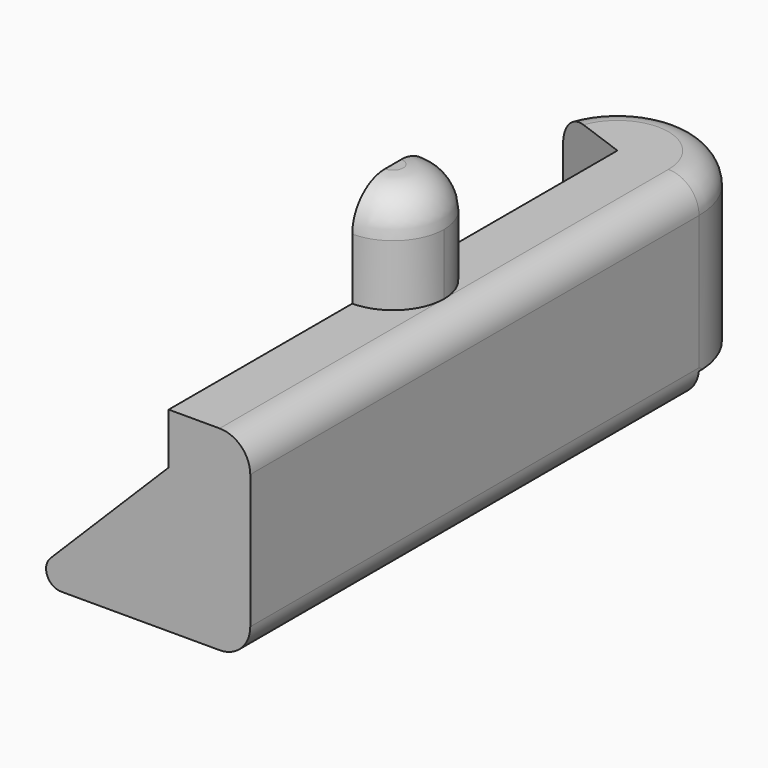
from build123d import *

# Parameters (mm, degrees)
F1_DEPTH      = 5.5
F3_DEPTH      = 1.14554
F4_T1_DEPTH   = 7
F5_R          = 0.15
F7_DEPTH      = 1.5
F7_DEPTH_BACK = 0.8
F8_T2_ANGLE   = 359.64
F9_DEPTH      = 0.5
F10_R         = 0.29999


# Not quite as in the source:
# - a fillet or chamfer that OpenCascade refuses, or shapes differently, is made with other operations: its cross-section is extruded or revolved along the edge and cut away or added
# - a fillet or chamfer is up to 0.001 mm smaller than in the source, because OpenCascade refuses the exact size


with BuildPart() as f1:
    # F0 (on Front) → F1 (new body)
    with BuildSketch(Plane.XZ):
        Polygon((1.0782154338, 1.8218530951), (0.2782154338, 1.8218530951), (-1.1359981286, 0.4076395328), (1.0782154338, 0.4076395328), align=None)
    extrude(amount=F1_DEPTH)

    # F2 (on face) → F3 (join)
    with BuildSketch(Plane.XY.offset(1.8218530951)):
        with BuildLine():
            Line((-0.4735386629, 0.2736161147), (0.2782154338, 0))
            Line((0.2782154338, 0), (1.0782154338, 0))
            ThreePointArc((1.0782154338, 0), (0.4171339759, 0.7878462024), (-0.4735386629, 0.2736161147))
        make_face()
    extrude(amount=-F3_DEPTH)

    # F4: fillet of radius 0.3 on 1 edges, made by hand

    # F4_s2 → F4_t1 (cut)
    with BuildSketch(Plane.XZ.offset(-0.75)):
        with BuildLine():
            ThreePointArc((1.0782154338, 0.7076395328), (0.9903474681, 0.4955074984), (0.7782154338, 0.4076395328))
            Line((0.7782154338, 0.4076395328), (1.0782154338, 0.4076395328))
            Line((1.0782154338, 0.4076395328), (1.0782154338, 0.7076395328))
        make_face()
    extrude(amount=F4_T1_DEPTH, mode=Mode.SUBTRACT)

    # F5
    f5_edges = [f1.edges().sort_by_distance(p)[0] for p in [
        (-1.135998, -2.75, 0.40764),
    ]]
    fillet(f5_edges, radius=F5_R)

    # F6 (on face) → F7 (join, two sides)
    with BuildSketch(Plane.XY.offset(1.8218530951)) as f7_sk:
        with BuildLine():
            ThreePointArc((0.2782154338, -3.25), (0.6317688243, -3.1035533906), (0.7782154338, -2.75))
            ThreePointArc((0.7782154338, -2.75), (0.6317688243, -2.3964466094), (0.2782154338, -2.25))
            Line((0.2782154338, -2.25), (0.2782154338, -3.25))
        make_face()
    extrude(amount=F7_DEPTH)
    extrude(f7_sk.sketch, amount=-F7_DEPTH_BACK)

    # F8: fillet of radius 0.4 on 1 edges, made by hand

    # F8_s1 → F8_t2 (revolve, cut)
    with BuildSketch(Plane(origin=(-0.0086365771, -2.7490988249, 0), x_dir=(0, 0, 1), z_dir=(-0.0031415875, -0.9999950652, 0))):
        with BuildLine():
            ThreePointArc((2.9218530951, 0.2131465736), (3.2046958076, 0.0959892861), (3.3218530951, -0.1868534264))
            Line((3.3218530951, -0.1868534264), (3.3218530951, 0.2131465736))
            Line((3.3218530951, 0.2131465736), (2.9218530951, 0.2131465736))
        make_face()
    revolve(axis=Axis((0.2782154338, -2.75, 3.3218530951), (0, 0, -1)), revolution_arc=F8_T2_ANGLE, mode=Mode.SUBTRACT)

    # F9 (add): faces of the model
    f9_faces = [f1.faces().sort_by_distance(p)[0] for p in [
        (0.632239132, -2.1810312273, 1.8218530951),
        (0.632239132, -2.1810312273, 1.8218530951),
    ]]
    extrude(f9_faces, amount=F9_DEPTH)

    # F10 (radius 0.3 in the source; OpenCascade refuses exactly that, so slightly less here)
    f10_edges = [f1.edges().sort_by_distance(p)[0] for p in [
        (1.078215, -2.75, 2.321853),
        (0.417134, 0.787846, 2.321853),
    ]]
    fillet(f10_edges, radius=F10_R)


solid = f1.part
